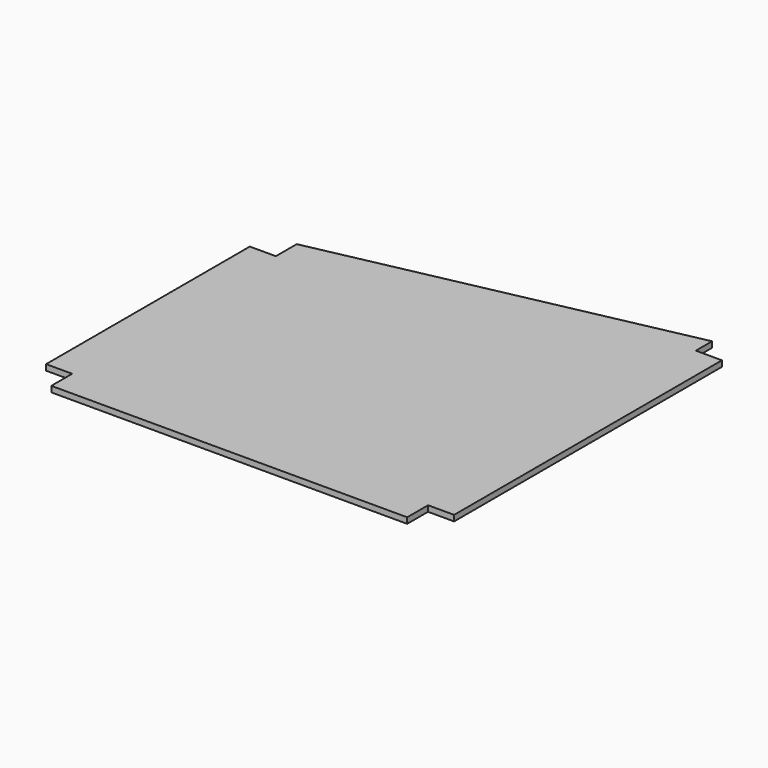
from build123d import *

# Parameters (mm, degrees)
F1_DEPTH = 12.7


# Not quite as in the source:
# - a length typed as a fraction of an inch, garbled in the dataset ("3 / 203.2 mm" for 3/8 in), is restored


with BuildPart() as f1:
    # F0 (on Top) → F1 (new body)
    with BuildSketch(Plane.XY):
        Polygon((57.15, 57.15), (57.15, 0), (831.85, 0), (837.0941968884, 0), (837.0941968884, 57.15), (894.2441968884, 57.15), (894.2441968884, 790.7659268673), (837.0941968884, 790.7659268673), (837.0941968884, 835.2612840102), (57.15, 672.3381097352), (57.15, 615.1881097352), (0, 615.1881097352), (0, 57.15), align=None)
    extrude(amount=F1_DEPTH)


solid = f1.part
